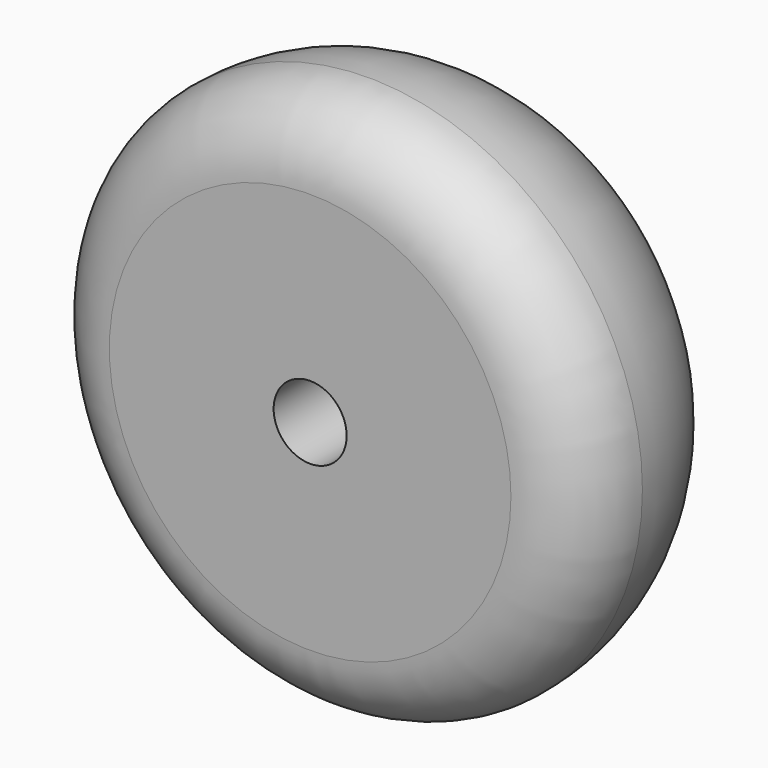
from build123d import *

# Parameters (mm, degrees)
F0_R     = 7.5
F0_R_2   = 1
F1_DEPTH = 7
F2_R     = 2
F3_R     = 4.99999


# Not quite as in the source:
# - a fillet or chamfer is up to 0.001 mm smaller than in the source, because OpenCascade refuses the exact size


with BuildPart() as f1:
    # F0 (on Front) → F1 (new body)
    with BuildSketch(Plane.XZ):
        Circle(F0_R)
        Circle(F0_R_2, mode=Mode.SUBTRACT)
    extrude(amount=F1_DEPTH)

    # F2
    f2_edges = [f1.edges().sort_by_distance(p)[0] for p in [
        (-7.5, -7, 0),
    ]]
    fillet(f2_edges, radius=F2_R)

    # F3 (radius 5 in the source; OpenCascade refuses exactly that, so slightly less here)
    f3_edges = [f1.edges().sort_by_distance(p)[0] for p in [
        (-7.5, 0, 0),
    ]]
    fillet(f3_edges, radius=F3_R)


solid = f1.part
